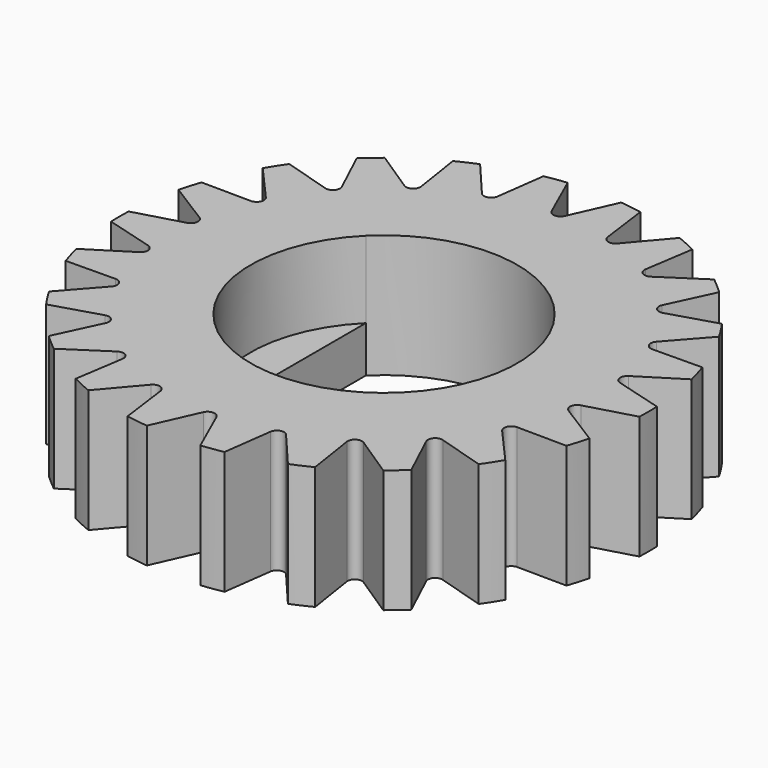
from build123d import *

# Parameters (mm, degrees)
F0_R            = 10.909800859
F1_DEPTH        = 5.08
F3_DEPTH        = 5.08
F3_COPIES_COUNT = 22
F4_R            = 5.5
F5_DEPTH        = 3.175


# Not quite as in the source:
# - a pattern or mirror of a feature is missing from the dataset's text; its kind, count and spacing are read off the source's solid


with BuildPart() as f1:
    # F0 (on Top) → F1 (new body)
    with BuildSketch(Plane.XY):
        Circle(F0_R)
        with BuildLine():
            ThreePointArc((3.8749986, -3.9031251389), (0, -5.5), (-3.8749986, -3.9031251389))
            Line((-3.8749986, -3.9031251389), (-3.8749986, 3.9031251389))
            ThreePointArc((-3.8749986, 3.9031251389), (0, 5.5), (3.8749986, 3.9031251389))
            Line((3.8749986, 3.9031251389), (3.8749986, -3.9031251389))
        make_face(mode=Mode.SUBTRACT)
    extrude(amount=F1_DEPTH)

    # F2 (on face) → F3 (cut, through all)
    with BuildSketch(Plane.XY.offset(5.08)):
        with BuildLine():
            Line((0.2718847261, 8.9821943232), (1.1039126824, 10.8538072386))
            ThreePointArc((1.1039126824, 10.8538072386), (0, 10.909800859), (-1.1039126824, 10.8538072386))
            Line((-1.1039126824, 10.8538072386), (-0.2718847261, 8.9821943232))
            ThreePointArc((-0.2718847261, 8.9821943232), (0, 8.8055210085), (0.2718847261, 8.9821943232))
        make_face()
    f3 = extrude(amount=-F3_DEPTH, mode=Mode.SUBTRACT)

    # F3_copies: F3 ×22 about axis
    f3_copies_axis = Axis((0, 0, 0), (0, 0, 1))
    for i in range(1, F3_COPIES_COUNT):
        add(f3.rotate(f3_copies_axis, i * 360 / F3_COPIES_COUNT), mode=Mode.SUBTRACT)

    # F4 (on face) → F5 (cut)
    with BuildSketch(Plane.XY.offset(5.08)):
        Circle(F4_R)
    extrude(amount=-F5_DEPTH, mode=Mode.SUBTRACT)


solid = f1.part
